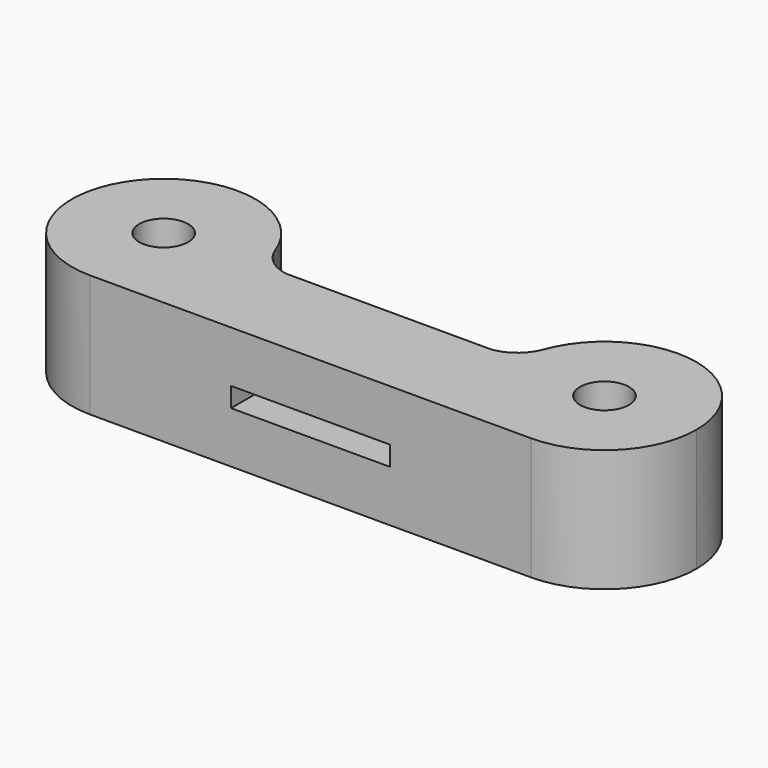
from build123d import *

# Parameters (mm, degrees)
F0_R     = 3.25
F0_R_2   = 1
F1_DEPTH = 5
F2_DEPTH = 3
F3_W     = 6.5
F3_H     = 0.8
F4_DEPTH = 25


with BuildPart() as f1:
    # F0 (on Top) → F1 (new body)
    with BuildSketch(Plane.XY):
        with BuildLine():
            ThreePointArc((-7.9180477187, -2.6999995224), (-5.2663972893, -1.6016499519), (-4.1680477187, 1.0500004776))
            ThreePointArc((-4.1680477187, 1.0500004776), (-4.1701339523, 1.1750700574), (-4.1763903319, 1.3000004776))
            ThreePointArc((-4.1763903319, 1.3000004776), (-4.2448197056, 1.8049150184), (-4.3810640575, 2.2958923592))
            ThreePointArc((-4.3810640575, 2.2958923592), (-10.9786517895, 3.2168421243), (-7.9180477187, -2.6999995224))
        make_face()
        with Locations((-7.9180477187, 1.0500004776)):
            Circle(F0_R, mode=Mode.SUBTRACT)
        with Locations((-7.9180477187, 1.0500004776)):
            Circle(F0_R)
        with Locations((-7.9180477187, 1.0500004776)):
            Circle(F0_R_2, mode=Mode.SUBTRACT)
        with BuildLine():
            ThreePointArc((6.3404704502, 1.3000004776), (7.3435150495, -1.5117372139), (10.082127837, -2.6999995224))
            ThreePointArc((10.082127837, -2.6999995224), (12.7337782665, -1.6016499519), (13.832127837, 1.0500004776))
            ThreePointArc((13.832127837, 1.0500004776), (10.7141133078, 4.7463627927), (6.5451441758, 2.2958923592))
            ThreePointArc((6.5451441758, 2.2958923592), (6.4088998239, 1.8049150184), (6.3404704502, 1.3000004776))
        make_face()
        with Locations((10.082127837, 1.0500004776)):
            Circle(F0_R, mode=Mode.SUBTRACT)
        with Locations((10.082127837, 1.0500004776)):
            Circle(F0_R)
        with Locations((10.082127837, 1.0500004776)):
            Circle(F0_R_2, mode=Mode.SUBTRACT)
        with BuildLine():
            ThreePointArc((-4.1763903319, 1.3000004776), (-4.1701339523, 1.1750700574), (-4.1680477187, 1.0500004776))
            ThreePointArc((-4.1680477187, 1.0500004776), (-5.2663972893, -1.6016499519), (-7.9180477187, -2.6999995224))
            Line((-7.9180477187, -2.6999995224), (10.082127837, -2.6999995224))
            ThreePointArc((10.082127837, -2.6999995224), (7.3435150495, -1.5117372139), (6.3404704502, 1.3000004776))
            Line((6.3404704502, 1.3000004776), (5.2561087846, 1.3000004776))
            Line((5.2561087846, 1.3000004776), (-3.0920286663, 1.3000004776))
            Line((-3.0920286663, 1.3000004776), (-4.1763903319, 1.3000004776))
        make_face()
        with BuildLine():
            ThreePointArc((-4.3810640575, 2.2958923592), (-4.2448197056, 1.8049150184), (-4.1763903319, 1.3000004776))
            Line((-4.1763903319, 1.3000004776), (-3.0920286663, 1.3000004776))
            ThreePointArc((-3.0920286663, 1.3000004776), (-3.8704928802, 1.6245723747), (-4.3810640575, 2.2958923592))
        make_face()
        with BuildLine():
            ThreePointArc((6.5451441758, 2.2958923592), (6.0345729985, 1.6245723747), (5.2561087846, 1.3000004776))
            Line((5.2561087846, 1.3000004776), (6.3404704502, 1.3000004776))
            ThreePointArc((6.3404704502, 1.3000004776), (6.4088998239, 1.8049150184), (6.5451441758, 2.2958923592))
        make_face()
    extrude(amount=F1_DEPTH)

    # F0 (on Top) → F2 (cut)
    with BuildSketch(Plane.XY):
        with Locations((10.082127837, 1.0500004776)):
            Circle(F0_R)
        with Locations((10.082127837, 1.0500004776)):
            Circle(F0_R_2, mode=Mode.SUBTRACT)
        with Locations((-7.9180477187, 1.0500004776)):
            Circle(F0_R)
        with Locations((-7.9180477187, 1.0500004776)):
            Circle(F0_R_2, mode=Mode.SUBTRACT)
    extrude(amount=F2_DEPTH, mode=Mode.SUBTRACT)

    # F3 (on face) → F4 (cut)
    with BuildSketch(Plane.XZ.offset(2.6999995224)):
        with Locations((1.0820400592, 2.5)):
            Rectangle(F3_W, F3_H)
    extrude(amount=-F4_DEPTH, mode=Mode.SUBTRACT)


solid = f1.part
